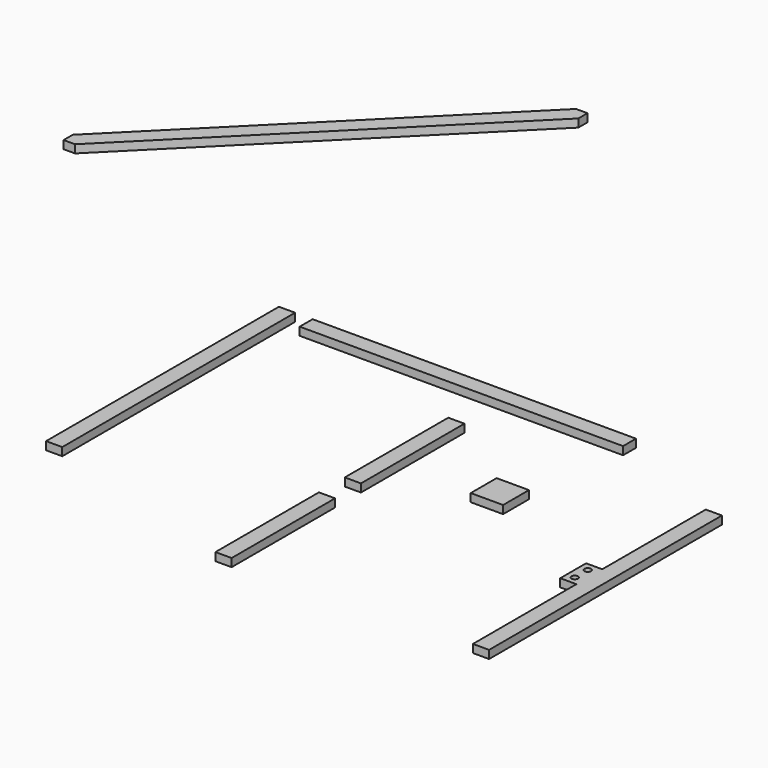
from build123d import *

# Parameters (mm, degrees)
F0_W      = 2000
F0_H      = 100
F1_DEPTH  = 50
F2_W      = 100
F2_H      = 1800
F3_DEPTH  = 50
F4_W      = 100
F4_H      = 800
F5_DEPTH  = 50
F6_R      = 20
F7_DEPTH  = 50
F9_DEPTH  = 50
F10_W     = 200
F10_H     = 200
F11_DEPTH = 50


# Not quite as in the source:
# - a feature names something its author has since deleted; it is built from what else it names


with BuildPart() as f1:
    # F0 (on Top) → F1 (new body)
    with BuildSketch(Plane.XY):
        with Locations((1000, -50)):
            Rectangle(F0_W, F0_H)
    extrude(amount=F1_DEPTH)


with BuildPart() as f3:
    # F2 (on Top) → F3 (new body)
    with BuildSketch(Plane.XY):
        with Locations((-158.4889411926, -900)):
            Rectangle(F2_W, F2_H)
    extrude(amount=F3_DEPTH)


with BuildPart() as f5:
    # F4 (on Top) → F5 (new body)
    with BuildSketch(Plane.XY):
        with Locations((1205.0287723541, -795.1983213425)):
            Rectangle(F4_W, F4_H)
    extrude(amount=F5_DEPTH)


with BuildPart() as f5b:
    # F4 (on Top) → F5, piece 2 (new body)
    with BuildSketch(Plane.XY):
        with Locations((1205.0287723541, -1795.1983213425)):
            Rectangle(F4_W, F4_H)
    extrude(amount=F5_DEPTH)


with BuildPart() as f7:
    # F6 (on Top) → F7 (new body)
    with BuildSketch(Plane.XY):
        Polygon((2826.1301040649, -2168.4369087219), (2826.1301040649, -368.4369087219), (2726.1301040649, -368.4369087219), (2726.1301040649, -1168.4369087219), (2626.1301040649, -1168.4369087219), (2626.1301040649, -1368.4369087219), (2726.1301040649, -1368.4369087219), (2726.1301040649, -2168.4369087219), align=None)
        with Locations((2676.1301040649, -1318.4369087219)):
            Circle(F6_R, mode=Mode.SUBTRACT)
        with Locations((2676.1301040649, -1218.4369087219)):
            Circle(F6_R, mode=Mode.SUBTRACT)
    extrude(amount=F7_DEPTH)


with BuildPart() as f9:
    # F8 (on Top) → F9 (new body)
    with BuildSketch(Plane.XY):
        Polygon((-2038.8407516299, 711.787879467), (-309.5514297485, 2441.0772013484), (-309.5514297485, 2511.787879467), (-380.2621078672, 2511.787879467), (-2109.5514297485, 782.4985575857), (-2109.5514297485, 711.787879467), align=None)
    extrude(amount=F9_DEPTH)


with BuildPart() as f11:
    # F10 (on Top) → F11 (new body)
    with BuildSketch(Plane.XY):
        with Locations((1832.345867157, -843.0387616158)):
            Rectangle(F10_W, F10_H)
    extrude(amount=F11_DEPTH)


solid = Compound([f1.part, f3.part, f5.part, f5b.part, f7.part, f9.part, f11.part])
